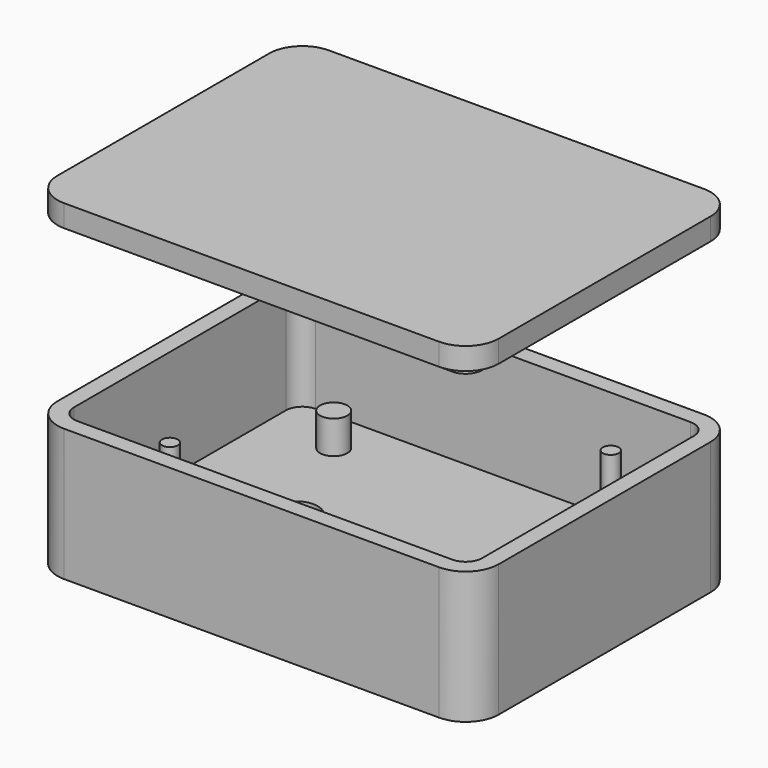
from build123d import *

# Parameters (mm, degrees)
F0_W      = 63.5
F0_H      = 47.625
F1_DEPTH  = 19.05
F2_R      = 4.7625
F4_DEPTH  = 15.875
F5_R      = 1.143
F6_DEPTH  = 12.7
F7_R      = 1.9685
F8_DEPTH  = 4.7625
F9_R      = 3.175
F10_DEPTH = 25.4
F13_DEPTH = 3.175
F15_DEPTH = 1.5875


with BuildPart() as f1:
    # F0 (on Top) → F1 (new body)
    with BuildSketch(Plane.XY):
        with Locations((31.75, 23.8125)):
            Rectangle(F0_W, F0_H)
    extrude(amount=F1_DEPTH)

    # F2
    f2_edges = [f1.edges().sort_by_distance(p)[0] for p in [
        (0, 0, 9.525),
        (63.5, 0, 9.525),
        (63.5, 47.625, 9.525),
        (0, 47.625, 9.525),
    ]]
    fillet(f2_edges, radius=F2_R)

    # F3 (on face) → F4 (cut)
    with BuildSketch(Plane.XY.offset(19.05)):
        with BuildLine():
            ThreePointArc((61.11875, 42.8625), (60.4212980227, 44.5462980227), (58.7375, 45.24375))
            Line((58.7375, 45.24375), (4.7625, 45.24375))
            ThreePointArc((4.7625, 45.24375), (3.0787019773, 44.5462980227), (2.38125, 42.8625))
            Line((2.38125, 42.8625), (2.38125, 4.7625))
            ThreePointArc((2.38125, 4.7625), (3.0787019773, 3.0787019773), (4.7625, 2.38125))
            Line((4.7625, 2.38125), (58.7375, 2.38125))
            ThreePointArc((58.7375, 2.38125), (60.4212980227, 3.0787019773), (61.11875, 4.7625))
            Line((61.11875, 4.7625), (61.11875, 42.8625))
        make_face()
    extrude(amount=-F4_DEPTH, mode=Mode.SUBTRACT)

    # F5 (on face) → F6 (join)
    with BuildSketch(Plane.XY.offset(3.175)):
        with Locations((12.319, 9.5885)):
            Circle(F5_R)
        with Locations((52.197, 39.0525)):
            Circle(F5_R)
    extrude(amount=F6_DEPTH)

    # F7 (on face) → F8 (join)
    with BuildSketch(Plane.XY.offset(3.175)):
        with Locations((12.319, 9.5885)):
            Circle(F7_R)
        with Locations((52.197, 39.0525)):
            Circle(F7_R)
        with Locations((12.319, 39.0525)):
            Circle(F7_R)
        with Locations((52.197, 9.5885)):
            Circle(F7_R)
    extrude(amount=F8_DEPTH)

    # F9 (on face) → F10 (cut)
    with BuildSketch(Plane.XY.offset(3.175)):
        with Locations((44.45, 23.8125)):
            Circle(F9_R)
        with Locations((19.05, 23.8125)):
            Circle(F9_R)
    extrude(amount=-F10_DEPTH, mode=Mode.SUBTRACT)


with BuildPart() as f13:
    # F12 (on offset) → F13 (new body)
    with BuildSketch(Plane.XY.offset(44.45)):
        with BuildLine():
            Line((0, 42.8625), (0, 4.7625))
            ThreePointArc((0, 4.7625), (1.3949039546, 1.3949039546), (4.7625, 0))
            Line((4.7625, 0), (58.7375, 0))
            ThreePointArc((58.7375, 0), (62.1050960454, 1.3949039546), (63.5, 4.7625))
            Line((63.5, 4.7625), (63.5, 42.8625))
            ThreePointArc((63.5, 42.8625), (62.1050960454, 46.2300960454), (58.7375, 47.625))
            Line((58.7375, 47.625), (4.7625, 47.625))
            ThreePointArc((4.7625, 47.625), (1.3949039546, 46.2300960454), (0, 42.8625))
        make_face()
    extrude(amount=F13_DEPTH)

    # F14 (on face) → F15 (join)
    with BuildSketch(Plane(origin=(0, 0, 44.45), x_dir=(1, 0, 0), z_dir=(0, 0, -1))):
        with BuildLine():
            Line((4.7625, -45.24375), (58.7375, -45.24375))
            ThreePointArc((58.7375, -45.24375), (60.4212980227, -44.5462980227), (61.11875, -42.8625))
            Line((61.11875, -42.8625), (61.11875, -4.7625))
            ThreePointArc((61.11875, -4.7625), (60.4212980227, -3.0787019773), (58.7375, -2.38125))
            Line((58.7375, -2.38125), (4.7625, -2.38125))
            ThreePointArc((4.7625, -2.38125), (3.0787019773, -3.0787019773), (2.38125, -4.7625))
            Line((2.38125, -4.7625), (2.38125, -42.8625))
            ThreePointArc((2.38125, -42.8625), (3.0787019773, -44.5462980227), (4.7625, -45.24375))
        make_face()
    extrude(amount=F15_DEPTH)


solid = Compound([f1.part, f13.part])
